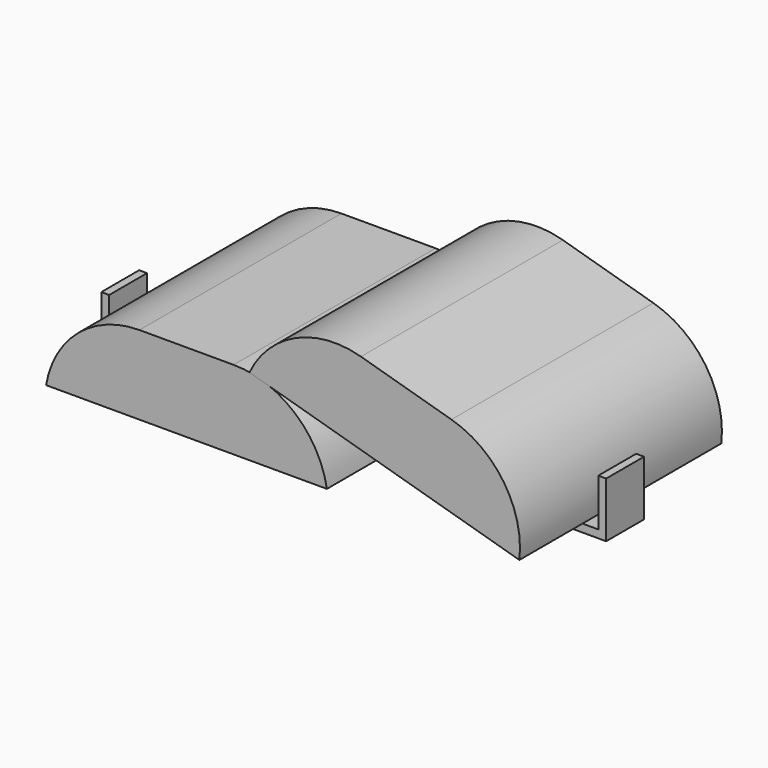
from build123d import *

# Parameters (mm, degrees)
F0_W        = 2.5
F0_H        = 15
F0_H_2      = 2.5
F1_DEPTH    = 15
F2_DEPTH    = 40
F3_T1_DEPTH = 227.9019945775
F4_DEPTH    = 40
F5_T1_DEPTH = 227.9019945775


# Not quite as in the source:
# - a fillet or chamfer that OpenCascade refuses, or shapes differently, is made with other operations: its cross-section is extruded or revolved along the edge and cut away or added


with BuildPart() as f1:
    # F0 (on Front) → F1 (new body)
    with BuildSketch(Plane.XZ):
        with Locations((-78.75, 10)):
            Rectangle(F0_W, F0_H)
        Polygon((-80, 2.5), (-80, 0), (77.5, 0), (77.5, 2.5), (72.5, 2.5), (11.5, 2.5), (-77.5, 2.5), align=None)
        with Locations((78.75, 1.25)):
            Rectangle(F0_W, F0_H_2)
        with Locations((78.75, 10)):
            Rectangle(F0_W, F0_H)
    extrude(amount=F1_DEPTH)


with BuildPart() as f2:
    # F0 (on Front) → F2 (new body, symmetric)
    with BuildSketch(Plane.XZ):
        Polygon((-77.5, 17.5), (-77.5, 2.5), (11.5, 2.5), (11.5, 19.9914685313), (-13.0522909385, 27.0317246677), (-12.9180151477, 27.5), (-77.5, 27.5), align=None)
        Polygon((-13.0522909385, 27.0317246677), (11.5, 19.9914685313), (11.5, 27.5), (-12.9180151477, 27.5), align=None)
    extrude(amount=F2_DEPTH, both=True)

    # F3: fillet of radius 30 on 2 edges, made by hand

    # F3_s2 → F3_t1 (cut)
    with BuildSketch(Plane.XZ.offset(-113.9509972888)):
        with BuildLine():
            ThreePointArc((-77.5, 2.5), (-67.2845178155, 20.4128784748), (-47.9196010845, 27.5))
            Line((-47.9196010845, 27.5), (-77.5, 27.5))
            Line((-77.5, 27.5), (-77.5, 2.5))
        make_face()
        with BuildLine():
            ThreePointArc((-18.0803989155, 27.5), (1.2845178155, 20.4128784748), (11.5, 2.5))
            Line((11.5, 2.5), (11.5, 27.5))
            Line((11.5, 27.5), (-18.0803989155, 27.5))
        make_face()
    extrude(amount=F3_T1_DEPTH, mode=Mode.SUBTRACT)


with BuildPart() as f4:
    # F0 (on Front) → F4 (new body, symmetric)
    with BuildSketch(Plane.XZ):
        Polygon((11.5, 19.9914685313), (72.5, 2.5), (79.3909338954, 26.5315423985), (-6.1613570431, 51.0632670662), (-12.9180151477, 27.5), (11.5, 27.5), align=None)
        Polygon((-13.0522909385, 27.0317246677), (11.5, 19.9914685313), (11.5, 27.5), (-12.9180151477, 27.5), align=None)
    extrude(amount=F4_DEPTH, both=True)

    # F5: fillet of radius 30 on 2 edges, made by hand

    # F5_s2 → F5_t1 (cut)
    with BuildSketch(Plane.XZ.offset(-113.9509972888)):
        with BuildLine():
            ThreePointArc((-13.0522909385, 27.0317246677), (1.7049192488, 41.4349201118), (22.273147385, 42.9098041251))
            Line((22.273147385, 42.9098041251), (-6.1613570431, 51.0632670662))
            Line((-6.1613570431, 51.0632670662), (-13.0522909385, 27.0317246677))
        make_face()
        with BuildLine():
            ThreePointArc((72.5, 2.5), (67.6177067284, 22.5347324395), (50.9564294674, 34.6850053395))
            Line((50.9564294674, 34.6850053395), (79.3909338954, 26.5315423985))
            Line((79.3909338954, 26.5315423985), (72.5, 2.5))
        make_face()
    extrude(amount=F5_T1_DEPTH, mode=Mode.SUBTRACT)


solid = Compound([f1.part, f2.part, f4.part])
